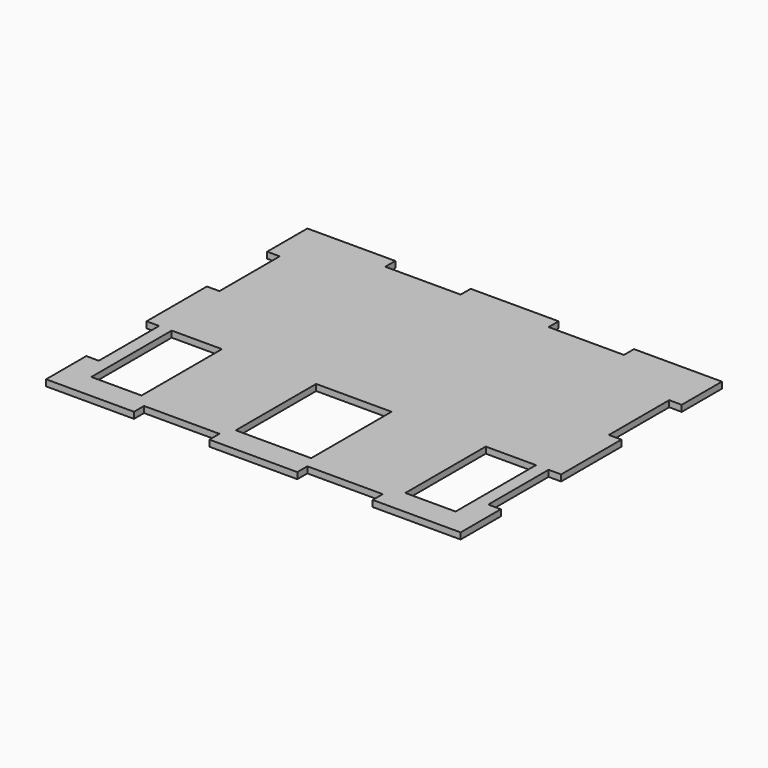
from build123d import *

# Parameters (mm, degrees)
F0_W     = 209.55
F0_H     = 165.1
F1_DEPTH = 3.175
F2_W     = 6.35
F2_H     = 38.1
F2_W_2   = 38.1
F2_H_2   = 6.35
F3_DEPTH = 25.4
F4_W     = 25.4
F4_H     = 50.8
F4_W_2   = 38.1
F5_DEPTH = 25.4


# Not quite as in the source:
# - a length typed as a fraction of an inch, garbled in the dataset ("3 / 203.2 mm" for 3/8 in), is restored


with BuildPart() as f1:
    # F0 (on Top) → F1 (new body)
    with BuildSketch(Plane.XY):
        Rectangle(F0_W, F0_H)
    extrude(amount=F1_DEPTH)

    # F2 (on face) → F3 (cut)
    with BuildSketch(Plane.XY.offset(3.175)):
        with Locations((-101.6, 38.1)):
            Rectangle(F2_W, F2_H)
        with Locations((-101.6, -38.1)):
            Rectangle(F2_W, F2_H)
        with Locations((101.6, 38.1)):
            Rectangle(F2_W, F2_H)
        with Locations((101.6, -38.1)):
            Rectangle(F2_W, F2_H)
        with Locations((-41.275, -79.375)):
            Rectangle(F2_W_2, F2_H_2)
        with Locations((41.275, -79.375)):
            Rectangle(F2_W_2, F2_H_2)
        with Locations((41.275, 79.375)):
            Rectangle(F2_W_2, F2_H_2)
        with Locations((-41.275, 79.375)):
            Rectangle(F2_W_2, F2_H_2)
    extrude(amount=-F3_DEPTH, mode=Mode.SUBTRACT)

    # F4 (on face) → F5 (cut)
    with BuildSketch(Plane.XY.offset(3.175)):
        with Locations((-79.375, -44.45)):
            Rectangle(F4_W, F4_H)
        with Locations((79.375, -44.45)):
            Rectangle(F4_W, F4_H)
        with Locations((0, -44.45)):
            Rectangle(F4_W_2, F4_H)
    extrude(amount=-F5_DEPTH, mode=Mode.SUBTRACT)


solid = f1.part
